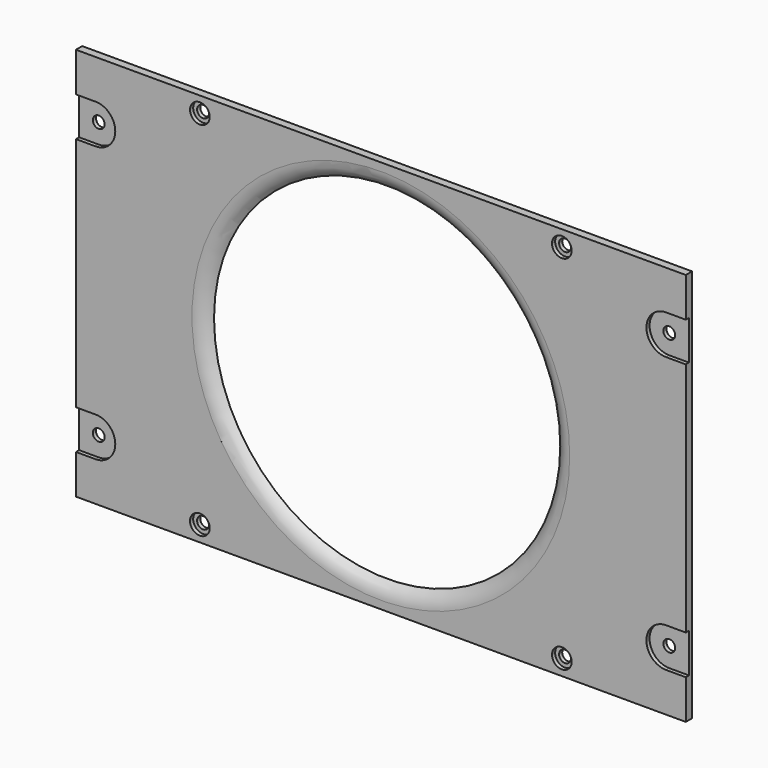
from build123d import *

# Parameters (mm, degrees)
F0_R     = 44
F1_DEPTH = 2
F0_R_2   = 1.5
F2_DEPTH = 1


# Not quite as in the source:
# - a fillet or chamfer that OpenCascade refuses, or shapes differently, is made with other operations: its cross-section is extruded or revolved along the edge and cut away or added


with BuildPart() as f1:
    # F0 (on Front) → F1 (new body)
    with BuildSketch(Plane.XZ):
        with BuildLine():
            Line((-77.5, -50), (77.5, -50))
            Line((77.5, -50), (77.5, -40))
            Line((77.5, -40), (72.5, -40))
            ThreePointArc((72.5, -40), (67.5, -35), (72.5, -30))
            Line((72.5, -30), (77.5, -30))
            Line((77.5, -30), (77.5, 30))
            Line((77.5, 30), (72.5, 30))
            ThreePointArc((72.5, 30), (67.5, 35), (72.5, 40))
            Line((72.5, 40), (77.5, 40))
            Line((77.5, 40), (77.5, 50))
            Line((77.5, 50), (-77.5, 50))
            Line((-77.5, 50), (-77.5, 40))
            Line((-77.5, 40), (-72.5, 40))
            ThreePointArc((-72.5, 40), (-67.5, 35), (-72.5, 30))
            Line((-72.5, 30), (-77.5, 30))
            Line((-77.5, 30), (-77.5, -30))
            Line((-77.5, -30), (-72.5, -30))
            ThreePointArc((-72.5, -30), (-67.5, -35), (-72.5, -40))
            Line((-72.5, -40), (-77.5, -40))
            Line((-77.5, -40), (-77.5, -50))
        make_face()
        with BuildLine():
            Line((43.5, -46), (-43.5, -46))
            ThreePointArc((-43.5, -46), (-47.767766953, -47.767766953), (-46, -43.5))
            Line((-46, -43.5), (-46, 43.5))
            ThreePointArc((-46, 43.5), (-47.767766953, 47.767766953), (-43.5, 46))
            Line((-43.5, 46), (43.5, 46))
            ThreePointArc((43.5, 46), (46, 48.5), (48.5, 46))
            ThreePointArc((48.5, 46), (47.767766953, 44.232233047), (46, 43.5))
            Line((46, 43.5), (46, -43.5))
            ThreePointArc((46, -43.5), (47.767766953, -44.232233047), (48.5, -46))
            ThreePointArc((48.5, -46), (46, -48.5), (43.5, -46))
        make_face(mode=Mode.SUBTRACT)
        with BuildLine():
            ThreePointArc((-46, -43.5), (-44.232233047, -44.232233047), (-43.5, -46))
            Line((-43.5, -46), (43.5, -46))
            ThreePointArc((43.5, -46), (44.232233047, -44.232233047), (46, -43.5))
            Line((46, -43.5), (46, 43.5))
            ThreePointArc((46, 43.5), (44.232233047, 44.232233047), (43.5, 46))
            Line((43.5, 46), (-43.5, 46))
            ThreePointArc((-43.5, 46), (-44.232233047, 44.232233047), (-46, 43.5))
            Line((-46, 43.5), (-46, -43.5))
        make_face()
        Circle(F0_R, mode=Mode.SUBTRACT)
    extrude(amount=F1_DEPTH)

    # F0 (on Front) → F2 (join)
    with BuildSketch(Plane.XZ):
        with BuildLine():
            Line((-77.5, -30), (-77.5, -40))
            Line((-77.5, -40), (-72.5, -40))
            ThreePointArc((-72.5, -40), (-67.5, -35), (-72.5, -30))
            Line((-72.5, -30), (-77.5, -30))
        make_face()
        with Locations((-72.5, -35)):
            Circle(F0_R_2, mode=Mode.SUBTRACT)
        with BuildLine():
            Line((-77.5, 40), (-77.5, 30))
            Line((-77.5, 30), (-72.5, 30))
            ThreePointArc((-72.5, 30), (-67.5, 35), (-72.5, 40))
            Line((-72.5, 40), (-77.5, 40))
        make_face()
        with Locations((-72.5, 35)):
            Circle(F0_R_2, mode=Mode.SUBTRACT)
        with BuildLine():
            Line((72.5, 30), (77.5, 30))
            Line((77.5, 30), (77.5, 40))
            Line((77.5, 40), (72.5, 40))
            ThreePointArc((72.5, 40), (67.5, 35), (72.5, 30))
        make_face()
        with Locations((72.5, 35)):
            Circle(F0_R_2, mode=Mode.SUBTRACT)
        with BuildLine():
            Line((72.5, -40), (77.5, -40))
            Line((77.5, -40), (77.5, -30))
            Line((77.5, -30), (72.5, -30))
            ThreePointArc((72.5, -30), (67.5, -35), (72.5, -40))
        make_face()
        with Locations((72.5, -35)):
            Circle(F0_R_2, mode=Mode.SUBTRACT)
        with BuildLine():
            ThreePointArc((-43.5, 46), (-47.767766953, 47.767766953), (-46, 43.5))
            Line((-46, 43.5), (-46, 44.5))
            ThreePointArc((-46, 44.5), (-47.0606601718, 47.0606601718), (-44.5, 46))
            Line((-44.5, 46), (-43.5, 46))
        make_face()
        with BuildLine():
            Line((-46, 44.5), (-46, 43.5))
            ThreePointArc((-46, 43.5), (-44.232233047, 44.232233047), (-43.5, 46))
            Line((-43.5, 46), (-44.5, 46))
            ThreePointArc((-44.5, 46), (-44.9393398282, 44.9393398282), (-46, 44.5))
        make_face()
        with BuildLine():
            Line((46, 44.5), (46, 43.5))
            ThreePointArc((46, 43.5), (47.767766953, 44.232233047), (48.5, 46))
            ThreePointArc((48.5, 46), (46, 48.5), (43.5, 46))
            Line((43.5, 46), (44.5, 46))
            ThreePointArc((44.5, 46), (46, 47.5), (47.5, 46))
            ThreePointArc((47.5, 46), (47.0606601718, 44.9393398282), (46, 44.5))
        make_face()
        with BuildLine():
            ThreePointArc((43.5, 46), (44.232233047, 44.232233047), (46, 43.5))
            Line((46, 43.5), (46, 44.5))
            ThreePointArc((46, 44.5), (44.9393398282, 44.9393398282), (44.5, 46))
            Line((44.5, 46), (43.5, 46))
        make_face()
        with BuildLine():
            Line((44.5, -46), (43.5, -46))
            ThreePointArc((43.5, -46), (46, -48.5), (48.5, -46))
            ThreePointArc((48.5, -46), (47.767766953, -44.232233047), (46, -43.5))
            Line((46, -43.5), (46, -44.5))
            ThreePointArc((46, -44.5), (47.0606601718, -44.9393398282), (47.5, -46))
            ThreePointArc((47.5, -46), (46, -47.5), (44.5, -46))
        make_face()
        with BuildLine():
            ThreePointArc((46, -43.5), (44.232233047, -44.232233047), (43.5, -46))
            Line((43.5, -46), (44.5, -46))
            ThreePointArc((44.5, -46), (44.9393398282, -44.9393398282), (46, -44.5))
            Line((46, -44.5), (46, -43.5))
        make_face()
        with BuildLine():
            Line((-44.5, -46), (-43.5, -46))
            ThreePointArc((-43.5, -46), (-44.232233047, -44.232233047), (-46, -43.5))
            Line((-46, -43.5), (-46, -44.5))
            ThreePointArc((-46, -44.5), (-44.9393398282, -44.9393398282), (-44.5, -46))
        make_face()
        with BuildLine():
            ThreePointArc((-46, -43.5), (-47.767766953, -47.767766953), (-43.5, -46))
            Line((-43.5, -46), (-44.5, -46))
            ThreePointArc((-44.5, -46), (-47.0606601718, -47.0606601718), (-46, -44.5))
            Line((-46, -44.5), (-46, -43.5))
        make_face()
    extrude(amount=F2_DEPTH)

    # F3: fillet of radius 5 on 1 edges, made by hand

    # F3_s1 → F3_t2 (revolve, cut)
    with BuildSketch(Plane.XY):
        with BuildLine():
            ThreePointArc((48, -2), (45.7639320225, -1.472135955), (44, 0))
            Line((44, 0), (44, -2))
            Line((44, -2), (48, -2))
        make_face()
    revolve(axis=Axis((0, -2, 0), (0, -1, 0)), mode=Mode.SUBTRACT)


solid = f1.part
